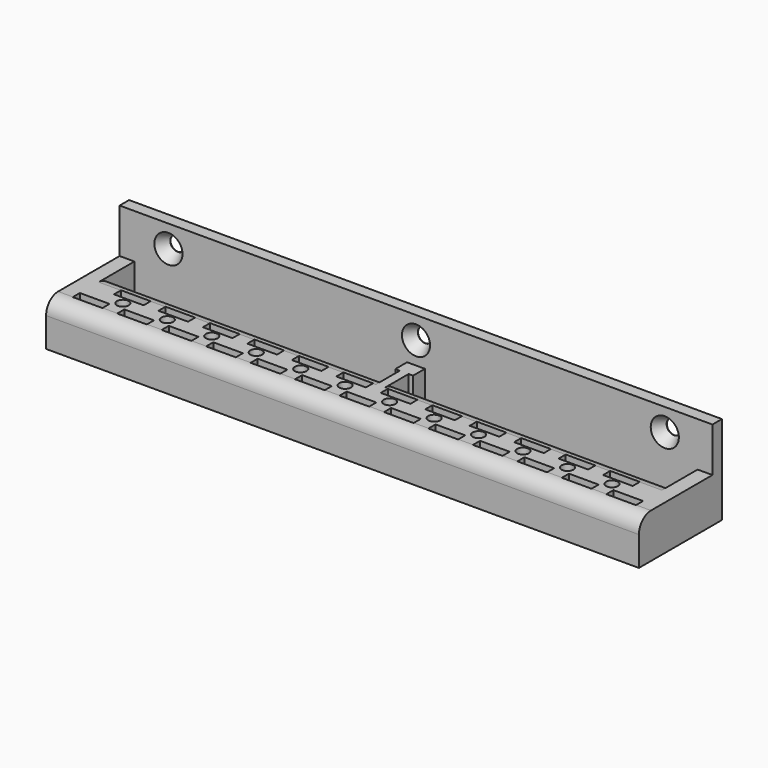
from build123d import *

# Parameters (mm, degrees)
F0_W           = 5
F0_H           = 5
F0_H_2         = 3
F0_W_2         = 10
F0_W_3         = 7.5
F0_R           = 2
F1_DEPTH       = 15
F2_W           = 5
F2_H           = 15
F2_W_2         = 3
F3_DEPTH       = 14
F4_W           = 5
F4_H           = 4
F4_W_2         = 92.004
F4_W_3         = 6
F4_W_4         = 91.996
F5_DEPTH       = 15
F5_DEPTH_BACK  = 15
F7_D           = 5
F7_DEPTH       = 20
F7_CSINK_D     = 9.5
F7_CSINK_ANGLE = 60
F7_TIP         = 1.5021515476
F8_W           = 1.5
F8_H           = 5
F9_DEPTH       = 15
F10_T1_DEPTH   = 200
F10_T3_DEPTH   = 93.496
F10_T5_DEPTH   = 93.504


# Not quite as in the source:
# - a fillet or chamfer that OpenCascade refuses, or shapes differently, is made with other operations: its cross-section is extruded or revolved along the edge and cut away or added


with BuildPart() as f1:
    # F0 (on Top) → F1 (new body)
    with BuildSketch(Plane.XY):
        with Locations((-98.9057382941, -13.6497081277)):
            Rectangle(F0_W, F0_H)
        Polygon((-86.4057382941, -11.1497081277), (-96.4057382941, -11.1497081277), (-96.4057382941, -16.1497081277), (-88.9057382941, -16.1497081277), (-86.4057382941, -16.1497081277), align=None)
        with Locations((-98.9057382941, -17.6497081277)):
            Rectangle(F0_W, F0_H_2)
        with Locations((-83.9057382941, -13.6497081277)):
            Rectangle(F0_W, F0_H)
        with Locations((-98.9057382941, -21.6497081277)):
            Rectangle(F0_W, F0_H)
        Polygon((-71.4057382941, -11.1497081277), (-81.4057382941, -11.1497081277), (-81.4057382941, -16.1497081277), (-78.9057382941, -16.1497081277), (-73.9057382941, -16.1497081277), (-71.4057382941, -16.1497081277), align=None)
        with Locations((-98.9057382941, -25.6497081277)):
            Rectangle(F0_W, F0_H_2)
        with Locations((-68.9057382941, -13.6497081277)):
            Rectangle(F0_W, F0_H)
        with Locations((-98.9057382941, -29.6497081277)):
            Rectangle(F0_W, F0_H)
        Polygon((-56.4057382941, -11.1497081277), (-66.4057382941, -11.1497081277), (-66.4057382941, -16.1497081277), (-63.9057382941, -16.1497081277), (-58.9057382941, -16.1497081277), (-56.4057382941, -16.1497081277), align=None)
        with Locations((-91.4057382941, -29.6497081277)):
            Rectangle(F0_W_2, F0_H)
        with Locations((-53.9057382941, -13.6497081277)):
            Rectangle(F0_W, F0_H)
        with Locations((-83.9057382941, -29.6497081277)):
            Rectangle(F0_W, F0_H)
        Polygon((-41.4057382941, -11.1497081277), (-51.4057382941, -11.1497081277), (-51.4057382941, -16.1497081277), (-48.9057382941, -16.1497081277), (-43.9057382941, -16.1497081277), (-41.4057382941, -16.1497081277), align=None)
        with Locations((-76.4057382941, -29.6497081277)):
            Rectangle(F0_W_2, F0_H)
        with Locations((-38.9057382941, -13.6497081277)):
            Rectangle(F0_W, F0_H)
        with Locations((-68.9057382941, -29.6497081277)):
            Rectangle(F0_W, F0_H)
        Polygon((-26.4057382941, -11.1497081277), (-36.4057382941, -11.1497081277), (-36.4057382941, -16.1497081277), (-33.9057382941, -16.1497081277), (-28.9057382941, -16.1497081277), (-26.4057382941, -16.1497081277), align=None)
        with Locations((-61.4057382941, -29.6497081277)):
            Rectangle(F0_W_2, F0_H)
        with Locations((-23.9057382941, -13.6497081277)):
            Rectangle(F0_W, F0_H)
        with Locations((-53.9057382941, -29.6497081277)):
            Rectangle(F0_W, F0_H)
        Polygon((-11.4057382941, -11.1497081277), (-21.4057382941, -11.1497081277), (-21.4057382941, -16.1497081277), (-18.9057382941, -16.1497081277), (-13.9057382941, -16.1497081277), (-11.4057382941, -16.1497081277), align=None)
        with Locations((-46.4057382941, -29.6497081277)):
            Rectangle(F0_W_2, F0_H)
        with Locations((-8.9057382941, -13.6497081277)):
            Rectangle(F0_W, F0_H)
        with Locations((-38.9057382941, -29.6497081277)):
            Rectangle(F0_W, F0_H)
        Polygon((3.5942617059, -11.1497081277), (-6.4057382941, -11.1497081277), (-6.4057382941, -16.1497081277), (-3.9057382941, -16.1497081277), (1.0942617059, -16.1497081277), (3.5942617059, -16.1497081277), align=None)
        with Locations((-31.4057382941, -29.6497081277)):
            Rectangle(F0_W_2, F0_H)
        with Locations((6.0942617059, -13.6497081277)):
            Rectangle(F0_W, F0_H)
        with Locations((-23.9057382941, -29.6497081277)):
            Rectangle(F0_W, F0_H)
        Polygon((18.5942617059, -11.1497081277), (8.5942617059, -11.1497081277), (8.5942617059, -16.1497081277), (11.0942617059, -16.1497081277), (16.0942617059, -16.1497081277), (18.5942617059, -16.1497081277), align=None)
        with Locations((-16.4057382941, -29.6497081277)):
            Rectangle(F0_W_2, F0_H)
        with Locations((21.0942617059, -13.6497081277)):
            Rectangle(F0_W, F0_H)
        with Locations((-8.9057382941, -29.6497081277)):
            Rectangle(F0_W, F0_H)
        Polygon((33.5942617059, -11.1497081277), (23.5942617059, -11.1497081277), (23.5942617059, -16.1497081277), (26.0942617059, -16.1497081277), (31.0942617059, -16.1497081277), (33.5942617059, -16.1497081277), align=None)
        with Locations((-1.4057382941, -29.6497081277)):
            Rectangle(F0_W_2, F0_H)
        with Locations((36.0942617059, -13.6497081277)):
            Rectangle(F0_W, F0_H)
        with Locations((6.0942617059, -29.6497081277)):
            Rectangle(F0_W, F0_H)
        Polygon((48.5942617059, -11.1497081277), (38.5942617059, -11.1497081277), (38.5942617059, -16.1497081277), (41.0942617059, -16.1497081277), (46.0942617059, -16.1497081277), (48.5942617059, -16.1497081277), align=None)
        with Locations((13.5942617059, -29.6497081277)):
            Rectangle(F0_W_2, F0_H)
        with Locations((51.0942617059, -13.6497081277)):
            Rectangle(F0_W, F0_H)
        with Locations((21.0942617059, -29.6497081277)):
            Rectangle(F0_W, F0_H)
        Polygon((63.5942617059, -11.1497081277), (53.5942617059, -11.1497081277), (53.5942617059, -16.1497081277), (56.0942617059, -16.1497081277), (61.0942617059, -16.1497081277), (63.5942617059, -16.1497081277), align=None)
        with Locations((28.5942617059, -29.6497081277)):
            Rectangle(F0_W_2, F0_H)
        with Locations((66.0942617059, -13.6497081277)):
            Rectangle(F0_W, F0_H)
        with Locations((36.0942617059, -29.6497081277)):
            Rectangle(F0_W, F0_H)
        Polygon((78.5942617059, -11.1497081277), (68.5942617059, -11.1497081277), (68.5942617059, -16.1497081277), (71.0942617059, -16.1497081277), (76.0942617059, -16.1497081277), (78.5942617059, -16.1497081277), align=None)
        with Locations((43.5942617059, -29.6497081277)):
            Rectangle(F0_W_2, F0_H)
        with Locations((81.0942617059, -13.6497081277)):
            Rectangle(F0_W, F0_H)
        with Locations((51.0942617059, -29.6497081277)):
            Rectangle(F0_W, F0_H)
        Polygon((93.5942617059, -11.1497081277), (83.5942617059, -11.1497081277), (83.5942617059, -16.1497081277), (86.0942617059, -16.1497081277), (91.0942617059, -16.1497081277), (93.5942617059, -16.1497081277), align=None)
        with Locations((58.5942617059, -29.6497081277)):
            Rectangle(F0_W_2, F0_H)
        with Locations((96.0942617059, -13.6497081277)):
            Rectangle(F0_W, F0_H)
        with Locations((66.0942617059, -29.6497081277)):
            Rectangle(F0_W, F0_H)
        with Locations((96.0942617059, -17.6497081277)):
            Rectangle(F0_W, F0_H_2)
        with Locations((73.5942617059, -29.6497081277)):
            Rectangle(F0_W_2, F0_H)
        with Locations((96.0942617059, -21.6497081277)):
            Rectangle(F0_W, F0_H)
        with Locations((81.0942617059, -29.6497081277)):
            Rectangle(F0_W, F0_H)
        with Locations((96.0942617059, -25.6497081277)):
            Rectangle(F0_W, F0_H_2)
        with Locations((88.5942617059, -29.6497081277)):
            Rectangle(F0_W_2, F0_H)
        with Locations((96.0942617059, -29.6497081277)):
            Rectangle(F0_W, F0_H)
        with Locations((-92.6557382941, -17.6497081277)):
            Rectangle(F0_W_3, F0_H_2)
        Polygon((-88.9057382941, -19.1497081277), (-96.4057382941, -19.1497081277), (-96.4057382941, -24.1497081277), (-86.4057382941, -24.1497081277), (-86.4057382941, -19.1497081277), align=None)
        Polygon((-81.4057382941, -19.1497081277), (-86.4057382941, -19.1497081277), (-86.4057382941, -24.1497081277), (-81.4057382941, -24.1497081277), (-81.4057382941, -21.6497081277), align=None)
        with Locations((-83.9057382941, -21.6497081277)):
            Circle(F0_R, mode=Mode.SUBTRACT)
        Polygon((-78.9057382941, -19.1497081277), (-81.4057382941, -19.1497081277), (-81.4057382941, -21.6497081277), (-81.4057382941, -24.1497081277), (-71.4057382941, -24.1497081277), (-71.4057382941, -21.6497081277), (-71.4057382941, -19.1497081277), (-73.9057382941, -19.1497081277), align=None)
        Polygon((-66.4057382941, -19.1497081277), (-71.4057382941, -19.1497081277), (-71.4057382941, -21.6497081277), (-71.4057382941, -24.1497081277), (-66.4057382941, -24.1497081277), align=None)
        with BuildLine():
            ThreePointArc((-66.9057382941, -21.6497081277), (-68.9057382941, -23.6497081277), (-70.9057382941, -21.6497081277))
            ThreePointArc((-70.9057382941, -21.6497081277), (-68.9057382941, -19.6497081277), (-66.9057382941, -21.6497081277))
        make_face(mode=Mode.SUBTRACT)
        Polygon((-63.9057382941, -19.1497081277), (-66.4057382941, -19.1497081277), (-66.4057382941, -24.1497081277), (-56.4057382941, -24.1497081277), (-56.4057382941, -19.1497081277), (-58.9057382941, -19.1497081277), align=None)
        with Locations((-53.9057382941, -21.6497081277)):
            Rectangle(F0_W, F0_H)
        with BuildLine():
            ThreePointArc((-51.9057382941, -21.6497081277), (-53.1403714294, -23.4974671927), (-55.3199518565, -23.0639216901))
            ThreePointArc((-55.3199518565, -23.0639216901), (-54.6711051589, -19.8019490627), (-51.9057382941, -21.6497081277))
        make_face(mode=Mode.SUBTRACT)
        Polygon((-48.9057382941, -19.1497081277), (-51.4057382941, -19.1497081277), (-51.4057382941, -24.1497081277), (-41.4057382941, -24.1497081277), (-41.4057382941, -19.1497081277), (-43.9057382941, -19.1497081277), align=None)
        with Locations((-38.9057382941, -21.6497081277)):
            Rectangle(F0_W, F0_H)
        with BuildLine():
            ThreePointArc((-36.9057382941, -21.6497081277), (-38.1403714294, -23.4974671927), (-40.3199518565, -23.0639216901))
            ThreePointArc((-40.3199518565, -23.0639216901), (-39.6711051589, -19.8019490627), (-36.9057382941, -21.6497081277))
        make_face(mode=Mode.SUBTRACT)
        Polygon((-33.9057382941, -19.1497081277), (-36.4057382941, -19.1497081277), (-36.4057382941, -24.1497081277), (-26.4057382941, -24.1497081277), (-26.4057382941, -21.6497081277), (-26.4057382941, -19.1497081277), (-28.9057382941, -19.1497081277), align=None)
        Polygon((-21.4057382941, -19.1497081277), (-26.4057382941, -19.1497081277), (-26.4057382941, -21.6497081277), (-26.4057382941, -24.1497081277), (-21.4057382941, -24.1497081277), align=None)
        with BuildLine():
            ThreePointArc((-21.9057382941, -21.6497081277), (-23.9057382941, -23.6497081277), (-25.9057382941, -21.6497081277))
            ThreePointArc((-25.9057382941, -21.6497081277), (-23.9057382941, -19.6497081277), (-21.9057382941, -21.6497081277))
        make_face(mode=Mode.SUBTRACT)
        Polygon((-18.9057382941, -19.1497081277), (-21.4057382941, -19.1497081277), (-21.4057382941, -24.1497081277), (-11.4057382941, -24.1497081277), (-11.4057382941, -21.6497081277), (-11.4057382941, -19.1497081277), (-13.9057382941, -19.1497081277), align=None)
        Polygon((-6.4057382941, -19.1497081277), (-11.4057382941, -19.1497081277), (-11.4057382941, -21.6497081277), (-11.4057382941, -24.1497081277), (-6.4057382941, -24.1497081277), align=None)
        with BuildLine():
            ThreePointArc((-6.9057382941, -21.6497081277), (-8.9057382941, -23.6497081277), (-10.9057382941, -21.6497081277))
            ThreePointArc((-10.9057382941, -21.6497081277), (-8.9057382941, -19.6497081277), (-6.9057382941, -21.6497081277))
        make_face(mode=Mode.SUBTRACT)
        Polygon((-3.9057382941, -19.1497081277), (-6.4057382941, -19.1497081277), (-6.4057382941, -24.1497081277), (3.5942617059, -24.1497081277), (3.5942617059, -19.1497081277), (1.0942617059, -19.1497081277), align=None)
        with Locations((6.0942617059, -21.6497081277)):
            Rectangle(F0_W, F0_H)
        with BuildLine():
            ThreePointArc((8.0942617059, -21.6497081277), (6.8596285706, -23.4974671927), (4.6800481435, -23.0639216901))
            ThreePointArc((4.6800481435, -23.0639216901), (5.3288948411, -19.8019490627), (8.0942617059, -21.6497081277))
        make_face(mode=Mode.SUBTRACT)
        Polygon((11.0942617059, -19.1497081277), (8.5942617059, -19.1497081277), (8.5942617059, -24.1497081277), (18.5942617059, -24.1497081277), (18.5942617059, -21.6497081277), (18.5942617059, -19.1497081277), (16.0942617059, -19.1497081277), align=None)
        Polygon((21.0942617059, -19.1497081277), (18.5942617059, -19.1497081277), (18.5942617059, -21.6497081277), (18.5942617059, -24.1497081277), (23.5942617059, -24.1497081277), (23.5942617059, -19.1497081277), align=None)
        with BuildLine():
            ThreePointArc((23.0942617059, -21.6497081277), (21.0942617059, -23.6497081277), (19.0942617059, -21.6497081277))
            ThreePointArc((19.0942617059, -21.6497081277), (21.0942617059, -19.6497081277), (23.0942617059, -21.6497081277))
        make_face(mode=Mode.SUBTRACT)
        Polygon((26.0942617059, -19.1497081277), (23.5942617059, -19.1497081277), (23.5942617059, -24.1497081277), (33.5942617059, -24.1497081277), (33.5942617059, -21.6497081277), (33.5942617059, -19.1497081277), (31.0942617059, -19.1497081277), align=None)
        Polygon((38.5942617059, -19.1497081277), (33.5942617059, -19.1497081277), (33.5942617059, -21.6497081277), (33.5942617059, -24.1497081277), (38.5942617059, -24.1497081277), align=None)
        with BuildLine():
            ThreePointArc((38.0942617059, -21.6497081277), (36.0942617059, -23.6497081277), (34.0942617059, -21.6497081277))
            ThreePointArc((34.0942617059, -21.6497081277), (36.0942617059, -19.6497081277), (38.0942617059, -21.6497081277))
        make_face(mode=Mode.SUBTRACT)
        Polygon((41.0942617059, -19.1497081277), (38.5942617059, -19.1497081277), (38.5942617059, -24.1497081277), (48.5942617059, -24.1497081277), (48.5942617059, -21.6497081277), (48.5942617059, -19.1497081277), (46.0942617059, -19.1497081277), align=None)
        Polygon((53.5942617059, -19.1497081277), (48.5942617059, -19.1497081277), (48.5942617059, -21.6497081277), (48.5942617059, -24.1497081277), (53.5942617059, -24.1497081277), align=None)
        with BuildLine():
            ThreePointArc((53.0942617059, -21.6497081277), (51.0942617059, -23.6497081277), (49.0942617059, -21.6497081277))
            ThreePointArc((49.0942617059, -21.6497081277), (51.0942617059, -19.6497081277), (53.0942617059, -21.6497081277))
        make_face(mode=Mode.SUBTRACT)
        Polygon((56.0942617059, -19.1497081277), (53.5942617059, -19.1497081277), (53.5942617059, -24.1497081277), (63.5942617059, -24.1497081277), (63.5942617059, -21.6497081277), (63.5942617059, -19.1497081277), (61.0942617059, -19.1497081277), align=None)
        Polygon((68.5942617059, -19.1497081277), (63.5942617059, -19.1497081277), (63.5942617059, -21.6497081277), (63.5942617059, -24.1497081277), (68.5942617059, -24.1497081277), align=None)
        with BuildLine():
            ThreePointArc((68.0942617059, -21.6497081277), (66.0942617059, -23.6497081277), (64.0942617059, -21.6497081277))
            ThreePointArc((64.0942617059, -21.6497081277), (66.0942617059, -19.6497081277), (68.0942617059, -21.6497081277))
        make_face(mode=Mode.SUBTRACT)
        Polygon((71.0942617059, -19.1497081277), (68.5942617059, -19.1497081277), (68.5942617059, -24.1497081277), (78.5942617059, -24.1497081277), (78.5942617059, -21.6497081277), (78.5942617059, -19.1497081277), (76.0942617059, -19.1497081277), align=None)
        Polygon((83.5942617059, -19.1497081277), (78.5942617059, -19.1497081277), (78.5942617059, -21.6497081277), (78.5942617059, -24.1497081277), (83.5942617059, -24.1497081277), align=None)
        with BuildLine():
            ThreePointArc((83.0942617059, -21.6497081277), (81.0942617059, -23.6497081277), (79.0942617059, -21.6497081277))
            ThreePointArc((79.0942617059, -21.6497081277), (81.0942617059, -19.6497081277), (83.0942617059, -21.6497081277))
        make_face(mode=Mode.SUBTRACT)
        Polygon((86.0942617059, -19.1497081277), (83.5942617059, -19.1497081277), (83.5942617059, -24.1497081277), (93.5942617059, -24.1497081277), (93.5942617059, -19.1497081277), align=None)
        with Locations((81.0942617059, -25.6497081277)):
            Rectangle(F0_W, F0_H_2)
        with Locations((66.0942617059, -25.6497081277)):
            Rectangle(F0_W, F0_H_2)
        with Locations((51.0942617059, -25.6497081277)):
            Rectangle(F0_W, F0_H_2)
        with Locations((36.0942617059, -25.6497081277)):
            Rectangle(F0_W, F0_H_2)
        with Locations((21.0942617059, -25.6497081277)):
            Rectangle(F0_W, F0_H_2)
        with Locations((6.0942617059, -25.6497081277)):
            Rectangle(F0_W, F0_H_2)
        with Locations((-8.9057382941, -25.6497081277)):
            Rectangle(F0_W, F0_H_2)
        with Locations((-23.9057382941, -25.6497081277)):
            Rectangle(F0_W, F0_H_2)
        with Locations((-38.9057382941, -25.6497081277)):
            Rectangle(F0_W, F0_H_2)
        with Locations((-53.9057382941, -25.6497081277)):
            Rectangle(F0_W, F0_H_2)
        with Locations((-68.9057382941, -25.6497081277)):
            Rectangle(F0_W, F0_H_2)
        with Locations((-83.9057382941, -25.6497081277)):
            Rectangle(F0_W, F0_H_2)
        with Locations((-76.4057382941, -17.6497081277)):
            Rectangle(F0_W, F0_H_2)
        with Locations((-61.4057382941, -17.6497081277)):
            Rectangle(F0_W, F0_H_2)
        with Locations((-46.4057382941, -17.6497081277)):
            Rectangle(F0_W, F0_H_2)
        with Locations((-31.4057382941, -17.6497081277)):
            Rectangle(F0_W, F0_H_2)
        with Locations((-16.4057382941, -17.6497081277)):
            Rectangle(F0_W, F0_H_2)
        with Locations((-1.4057382941, -17.6497081277)):
            Rectangle(F0_W, F0_H_2)
        with Locations((13.5942617059, -17.6497081277)):
            Rectangle(F0_W, F0_H_2)
        with Locations((28.5942617059, -17.6497081277)):
            Rectangle(F0_W, F0_H_2)
        with Locations((43.5942617059, -17.6497081277)):
            Rectangle(F0_W, F0_H_2)
        with Locations((58.5942617059, -17.6497081277)):
            Rectangle(F0_W, F0_H_2)
        with Locations((73.5942617059, -17.6497081277)):
            Rectangle(F0_W, F0_H_2)
        Polygon((93.5942617059, -19.1497081277), (93.5942617059, -16.1497081277), (91.0942617059, -16.1497081277), (86.0942617059, -16.1497081277), (86.0942617059, -19.1497081277), align=None)
    extrude(amount=F1_DEPTH)

    # F2 (on face) → F3 (join)
    with BuildSketch(Plane(origin=(0, -11.1497081277, 0), x_dir=(-1, 0, 0), z_dir=(0, 1, 0))):
        with Locations((-96.0942617059, 7.5)):
            Rectangle(F2_W, F2_H)
        with Locations((-0.0902617059, 7.5)):
            Rectangle(F2_W_2, F2_H)
        with Locations((2.9097382941, 7.5)):
            Rectangle(F2_W_2, F2_H)
        with Locations((98.9057382941, 7.5)):
            Rectangle(F2_W, F2_H)
    extrude(amount=F3_DEPTH)

    # F4 (on face) → F5 (join, two sides)
    with BuildSketch(Plane.XY.offset(15)) as f5_sk:
        with Locations((96.0942617059, 0.8502918723)):
            Rectangle(F4_W, F4_H)
        with Locations((47.5922617059, 0.8502918723)):
            Rectangle(F4_W_2, F4_H)
        with Locations((-1.4097382941, 0.8502918723)):
            Rectangle(F4_W_3, F4_H)
        with Locations((-50.4077382941, 0.8502918723)):
            Rectangle(F4_W_4, F4_H)
        with Locations((-98.9057382941, 0.8502918723)):
            Rectangle(F4_W, F4_H)
    extrude(amount=F5_DEPTH)
    extrude(f5_sk.sketch, amount=-F5_DEPTH_BACK)

    # F7
    with Locations(Plane.XZ.offset(1.1497081277)):
        with Locations((-1.4097382941, 22.5), (82.5222954154, 22.5), (-84.9269106984, 22.5)):
            CounterSinkHole(F7_D / 2, F7_CSINK_D / 2, depth=F7_DEPTH, counter_sink_angle=F7_CSINK_ANGLE)
            with Locations((0, 0, -(F7_DEPTH + F7_TIP / 2))):  # 118° drill point
                Cone(0, F7_D / 2, F7_TIP, mode=Mode.SUBTRACT)

    # F8 (on face) → F9 (cut)
    with BuildSketch(Plane.XY.offset(15)):
        with Locations((-3.6597382941, -8.6497081277)):
            Rectangle(F8_W, F8_H)
        with Locations((0.8402617059, -8.6497081277)):
            Rectangle(F8_W, F8_H)
    extrude(amount=-F9_DEPTH, mode=Mode.SUBTRACT)

    # F10: fillet of radius 5.08 on 3 edges, made by hand

    # F10_s2 → F10_t1 (cut)
    with BuildSketch(Plane.YZ.offset(-101.4057382941)):
        with BuildLine():
            ThreePointArc((-27.0697081277, 15), (-30.6618105761, 13.5121024484), (-32.1497081277, 9.92))
            Line((-32.1497081277, 9.92), (-32.2513081277, 9.92))
            Line((-32.2513081277, 9.92), (-32.2513081277, 15.1016))
            Line((-32.2513081277, 15.1016), (-27.0697081277, 15.1016))
            Line((-27.0697081277, 15.1016), (-27.0697081277, 15))
        make_face()
    extrude(amount=F10_T1_DEPTH, mode=Mode.SUBTRACT)

    # F10_s4 → F10_t3 (cut)
    with BuildSketch(Plane.YZ.offset(-96.4057382941)):
        with BuildLine():
            ThreePointArc((-16.2297081277, 15), (-12.6376056793, 13.5121024484), (-11.1497081277, 9.92))
            Line((-11.1497081277, 9.92), (-11.0481081277, 9.92))
            Line((-11.0481081277, 9.92), (-11.0481081277, 15.1016))
            Line((-11.0481081277, 15.1016), (-16.2297081277, 15.1016))
            Line((-16.2297081277, 15.1016), (-16.2297081277, 15))
        make_face()
    extrude(amount=F10_T3_DEPTH, mode=Mode.SUBTRACT)

    # F10_s6 → F10_t5 (cut)
    with BuildSketch(Plane.YZ.offset(0.0902617059)):
        with BuildLine():
            ThreePointArc((-16.2297081277, 15), (-12.6376056793, 13.5121024484), (-11.1497081277, 9.92))
            Line((-11.1497081277, 9.92), (-11.0481081277, 9.92))
            Line((-11.0481081277, 9.92), (-11.0481081277, 15.1016))
            Line((-11.0481081277, 15.1016), (-16.2297081277, 15.1016))
            Line((-16.2297081277, 15.1016), (-16.2297081277, 15))
        make_face()
    extrude(amount=F10_T5_DEPTH, mode=Mode.SUBTRACT)


solid = f1.part
